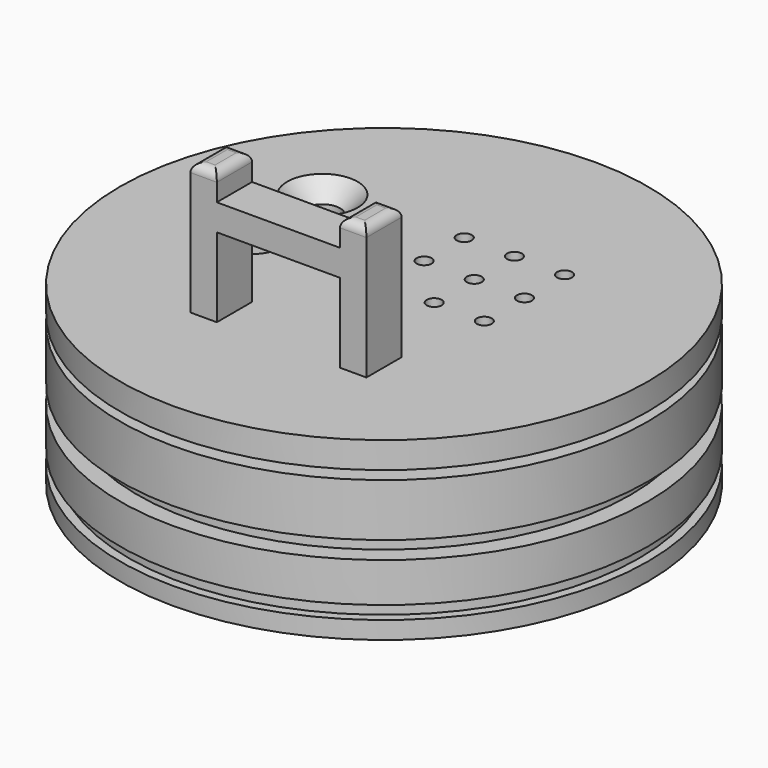
from build123d import *

# Parameters (mm, degrees)
F2_R           = 0.85
F3_DEPTH       = 10
F2_W           = 3
F2_H           = 5
F4_DEPTH       = 15
F6_R           = 1
F7_D           = 4
F7_CBORE_D     = 7.2
F7_CBORE_DEPTH = 3.9
F8_D           = 4
F8_DEPTH       = 20
F8_CSINK_D     = 8
F8_CSINK_ANGLE = 90
F8_TIP         = 1.2017212381
F5_W           = 5
F5_H           = 3
F9_DEPTH       = 14


# Not quite as in the source:
# - a feature of the source that left no trace in its solid (it failed there, or was rolled back) is left out


with BuildPart() as f1:
    # F0 (on Front) → F1 (revolve)
    with BuildSketch(Plane.XZ):
        Polygon((0, 22.0396561921), (-30, 22.0396561921), (-30, 2.0396561921), (0, 2.0396561921), (0, 4.0396561921), (-1, 4.0396561921), (-1, 5.5396561921), (0, 5.5396561921), (0, 10.0396561921), (-2, 10.0396561921), (-2, 12.0396561921), (0, 12.0396561921), (0, 18.0396561921), (-3, 18.0396561921), (-3, 19.0396561921), (0, 19.0396561921), align=None)
    revolve(axis=Axis((-30, 0, 12.0396561921), (0, 0, -1)))

    # F2 (on face) → F3 (cut)
    with BuildSketch(Plane.XY.offset(22.0396561921)):
        with BuildLine():
            ThreePointArc((-30.85, 0), (-30, -0.85), (-29.15, 0))
            ThreePointArc((-29.15, 0), (-30, 0.85), (-30.85, 0))
        make_face()
        with Locations((-30, 5.7)):
            Circle(F2_R)
        with Locations((-30, 11.4)):
            Circle(F2_R)
        with Locations((-24.3, 0)):
            Circle(F2_R)
        with Locations((-24.3, 5.7)):
            Circle(F2_R)
        with Locations((-24.3, 11.4)):
            Circle(F2_R)
        with Locations((-18.6, 0)):
            Circle(F2_R)
        with Locations((-18.6, 5.7)):
            Circle(F2_R)
        with Locations((-18.6, 11.4)):
            Circle(F2_R)
    extrude(amount=-F3_DEPTH, mode=Mode.SUBTRACT)

    # F2 (on face) → F4 (join)
    with BuildSketch(Plane.XY.offset(22.0396561921)):
        with Locations((-21.5, -12.5)):
            Rectangle(F2_W, F2_H)
        with Locations((-38.5, -12.5)):
            Rectangle(F2_W, F2_H)
    extrude(amount=F4_DEPTH)

    # F6
    f6_edges = [f1.edges().sort_by_distance(p)[0] for p in [
        (-38.5, -10, 37.039656),
        (-40, -12.5, 37.039656),
        (-38.5, -15, 37.039656),
        (-37, -12.5, 37.039656),
        (-23, -12.5, 37.039656),
        (-21.5, -15, 37.039656),
        (-20, -12.5, 37.039656),
        (-21.5, -10, 37.039656),
    ]]
    fillet(f6_edges, radius=F6_R)

    # F7 (through all)
    with Locations(Plane.XY.offset(22.0396561921)):
        with Locations((-45, 0)):
            CounterBoreHole(F7_D / 2, F7_CBORE_D / 2, F7_CBORE_DEPTH)

    # F8
    with Locations(Plane.XY.offset(22.0396561921)):
        with Locations((-45, 10)):
            CounterSinkHole(F8_D / 2, F8_CSINK_D / 2, depth=F8_DEPTH, counter_sink_angle=F8_CSINK_ANGLE)
            with Locations((0, 0, -(F8_DEPTH + F8_TIP / 2))):  # 118° drill point
                Cone(0, F8_D / 2, F8_TIP, mode=Mode.SUBTRACT)

    # F5 (on face) → F9 (join)
    with BuildSketch(Plane.YZ.offset(-37)):
        with Locations((-12.5, 32.5396561921)):
            Rectangle(F5_W, F5_H)
    extrude(amount=F9_DEPTH)


solid = f1.part
